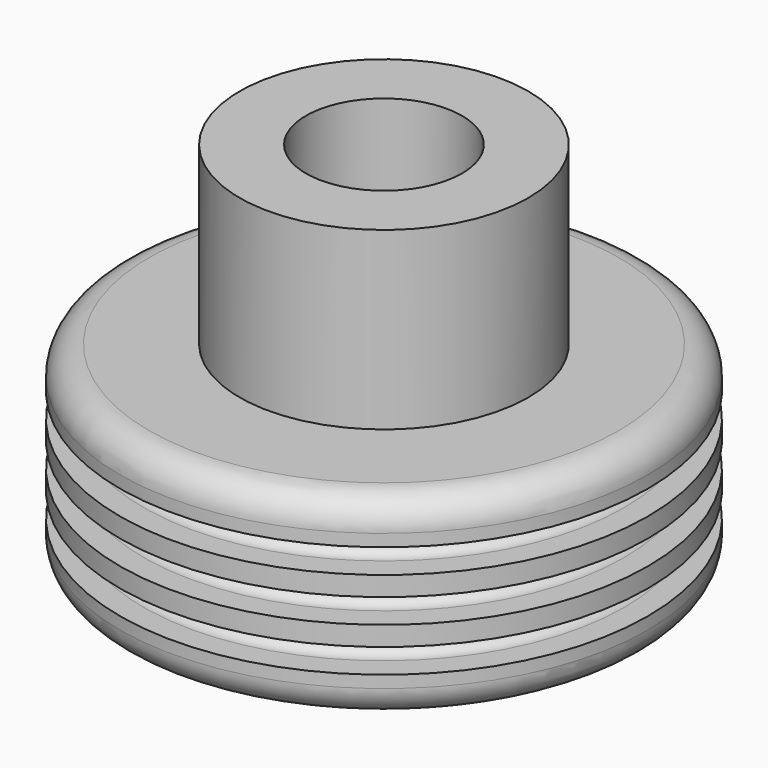
from build123d import *

# Parameters (mm, degrees)
F0_R     = 13.525
F0_R_2   = 4
F1_DEPTH = 19
F2_R     = 6.5
F3_DEPTH = 3
F4_R     = 13.525
F4_R_2   = 7.4
F5_DEPTH = 9
F6_R     = 1.5


# Not quite as in the source:
# - a feature names something its author has since deleted; it is built from what else it names


with BuildPart() as f1:
    # F0 (on Top) → F1 (new body)
    with BuildSketch(Plane.XY):
        Circle(F0_R)
        Circle(F0_R_2, mode=Mode.SUBTRACT)
    extrude(amount=F1_DEPTH)

    # F2 (on face) → F3 (cut)
    with BuildSketch(Plane(origin=(0, 0, 0), x_dir=(1, 0, 0), z_dir=(0, 0, -1))):
        Circle(F2_R)
    extrude(amount=-F3_DEPTH, mode=Mode.SUBTRACT)

    # F4 (on face) → F5 (cut)
    with BuildSketch(Plane.XY.offset(19)):
        Circle(F4_R)
        Circle(F4_R_2, mode=Mode.SUBTRACT)
    extrude(amount=-F5_DEPTH, mode=Mode.SUBTRACT)

    # F6
    f6_edges = [f1.edges().sort_by_distance(p)[0] for p in [
        (-13.525, 0, 10),
        (-13.525, 0, 0),
    ]]
    fillet(f6_edges, radius=F6_R)

    # F7 (on Right) → F8 (revolve, cut)
    with BuildSketch(Plane.YZ):
        with BuildLine():
            ThreePointArc((-12.3118543997, 2.125), (-11.6868543997, 2.75), (-12.3118543997, 3.375))
            Line((-12.3118543997, 3.375), (-14.8118543997, 3.375))
            Line((-14.8118543997, 3.375), (-14.8118543997, 2.75))
            Line((-14.8118543997, 2.75), (-14.8118543997, 2.125))
            Line((-14.8118543997, 2.125), (-12.3118543997, 2.125))
        make_face()
        with BuildLine():
            Line((-17.3118543997, 6.625), (-14.8118543997, 6.625))
            Line((-14.8118543997, 6.625), (-12.3118543997, 6.625))
            ThreePointArc((-12.3118543997, 6.625), (-11.6868543997, 7.25), (-12.3118543997, 7.875))
            Line((-12.3118543997, 7.875), (-17.3118543997, 7.875))
            Line((-17.3118543997, 7.875), (-17.3118543997, 6.625))
        make_face()
        Polygon((-17.3118543997, 4.375), (-14.8118543997, 4.375), (-14.8118543997, 5), (-14.8118543997, 5.625), (-17.3118543997, 5.625), align=None)
        with BuildLine():
            Line((-14.8118543997, 5), (-14.8118543997, 4.375))
            Line((-14.8118543997, 4.375), (-12.3118543997, 4.375))
            ThreePointArc((-12.3118543997, 4.375), (-11.6868543997, 5), (-12.3118543997, 5.625))
            Line((-12.3118543997, 5.625), (-14.8118543997, 5.625))
            Line((-14.8118543997, 5.625), (-14.8118543997, 5))
        make_face()
        Polygon((-14.8118543997, 2.75), (-14.8118543997, 3.375), (-17.3118543997, 3.375), (-17.3118543997, 2.125), (-14.8118543997, 2.125), align=None)
    revolve(axis=Axis((0, 0, 10.2130547166), (0, 0, 1)), mode=Mode.SUBTRACT)


solid = f1.part
